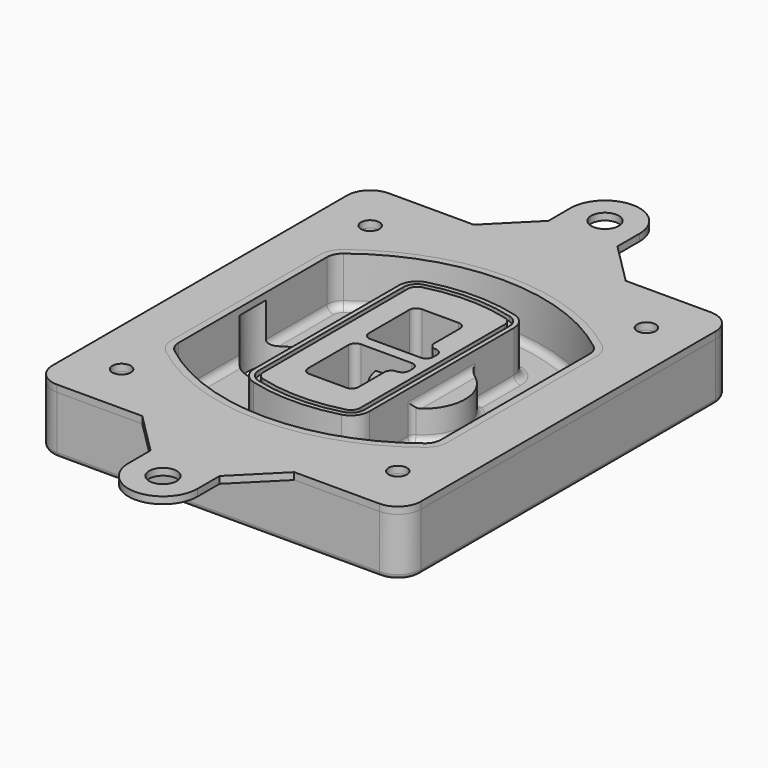
from build123d import *

# Parameters (mm, degrees)
F0_R      = 4
F1_DEPTH  = 25
F2_DEPTH  = 3
F3_DEPTH  = 18
F5_DEPTH  = 21
F6_DEPTH  = 2
F8_DEPTH  = 20
F9_DEPTH  = 16
F10_DEPTH = 25
F7_R      = 6
F7_R_2    = 4
F11_DEPTH = 6
F13_DEPTH = 9
F14_R     = 3
F15_R     = 2
F16_R     = 4
F16_R_2   = 6
F17_DEPTH = 3


with BuildPart() as f1:
    # F0 (on Top) → F1 (new body)
    with BuildSketch(Plane.XY):
        with BuildLine():
            ThreePointArc((-80, -80), (-77.0710678119, -87.0710678119), (-70, -90))
            Line((-70, -90), (70, -90))
            ThreePointArc((70, -90), (77.0710678119, -87.0710678119), (80, -80))
            Line((80, -80), (80, 80))
            ThreePointArc((80, 80), (77.0710678119, 87.0710678119), (70, 90))
            Line((70, 90), (-70, 90))
            ThreePointArc((-70, 90), (-77.0710678119, 87.0710678119), (-80, 80))
            Line((-80, 80), (-80, -80))
        make_face()
        with Locations((-60, -67.5)):
            Circle(F0_R, mode=Mode.SUBTRACT)
        with Locations((-60, 67.5)):
            Circle(F0_R, mode=Mode.SUBTRACT)
        with Locations((60, -67.5)):
            Circle(F0_R, mode=Mode.SUBTRACT)
        with BuildLine():
            ThreePointArc((-64, 40.2934422872), (-62.5820384798, 46.4328484224), (-58.6153846154, 51.3286200352))
            ThreePointArc((-58.6153846154, 51.3286200352), (0, 71.5), (58.6153846154, 51.3286200352))
            ThreePointArc((58.6153846154, 51.3286200352), (62.5820384798, 46.4328484224), (64, 40.2934422872))
            Line((64, 40.2934422872), (64, -40.2934422872))
            ThreePointArc((64, -40.2934422872), (62.5820384798, -46.4328484224), (58.6153846154, -51.3286200352))
            ThreePointArc((58.6153846154, -51.3286200352), (0, -71.5), (-58.6153846154, -51.3286200352))
            ThreePointArc((-58.6153846154, -51.3286200352), (-62.5820384798, -46.4328484224), (-64, -40.2934422872))
            Line((-64, -40.2934422872), (-64, 40.2934422872))
        make_face(mode=Mode.SUBTRACT)
        with Locations((60, 67.5)):
            Circle(F0_R, mode=Mode.SUBTRACT)
        with BuildLine():
            ThreePointArc((58.6153846154, 51.3286200352), (0, 71.5), (-58.6153846154, 51.3286200352))
            ThreePointArc((-58.6153846154, 51.3286200352), (-62.5820384798, 46.4328484224), (-64, 40.2934422872))
            Line((-64, 40.2934422872), (-64, -40.2934422872))
            ThreePointArc((-64, -40.2934422872), (-62.5820384798, -46.4328484224), (-58.6153846154, -51.3286200352))
            ThreePointArc((-58.6153846154, -51.3286200352), (0, -71.5), (58.6153846154, -51.3286200352))
            ThreePointArc((58.6153846154, -51.3286200352), (62.5820384798, -46.4328484224), (64, -40.2934422872))
            Line((64, -40.2934422872), (64, 40.2934422872))
            ThreePointArc((64, 40.2934422872), (62.5820384798, 46.4328484224), (58.6153846154, 51.3286200352))
        make_face()
        with BuildLine():
            Line((-60, -40.2934422872), (-60, 40.2934422872))
            ThreePointArc((-60, 40.2934422872), (-58.9871703427, 44.6787323838), (-56.1538461538, 48.1757121072))
            ThreePointArc((-56.1538461538, 48.1757121072), (0, 67.5), (56.1538461538, 48.1757121072))
            ThreePointArc((56.1538461538, 48.1757121072), (58.9871703427, 44.6787323838), (60, 40.2934422872))
            Line((60, 40.2934422872), (60, -40.2934422872))
            ThreePointArc((60, -40.2934422872), (58.9871703427, -44.6787323838), (56.1538461538, -48.1757121072))
            ThreePointArc((56.1538461538, -48.1757121072), (0, -67.5), (-56.1538461538, -48.1757121072))
            ThreePointArc((-56.1538461538, -48.1757121072), (-58.9871703427, -44.6787323838), (-60, -40.2934422872))
        make_face(mode=Mode.SUBTRACT)
        with BuildLine():
            ThreePointArc((-56.1538461538, 48.1757121072), (-58.9871703427, 44.6787323838), (-60, 40.2934422872))
            Line((-60, 40.2934422872), (-60, -40.2934422872))
            ThreePointArc((-60, -40.2934422872), (-58.9871703427, -44.6787323838), (-56.1538461538, -48.1757121072))
            ThreePointArc((-56.1538461538, -48.1757121072), (0, -67.5), (56.1538461538, -48.1757121072))
            ThreePointArc((56.1538461538, -48.1757121072), (58.9871703427, -44.6787323838), (60, -40.2934422872))
            Line((60, -40.2934422872), (60, 40.2934422872))
            ThreePointArc((60, 40.2934422872), (58.9871703427, 44.6787323838), (56.1538461538, 48.1757121072))
            ThreePointArc((56.1538461538, 48.1757121072), (0, 67.5), (-56.1538461538, 48.1757121072))
        make_face()
        with BuildLine():
            ThreePointArc((54.3076923077, 45.8110311612), (56.2910192399, 43.3631453548), (57, 40.2934422872))
            Line((57, 40.2934422872), (57, -40.2934422872))
            ThreePointArc((57, -40.2934422872), (56.2910192399, -43.3631453548), (54.3076923077, -45.8110311612))
            ThreePointArc((54.3076923077, -45.8110311612), (0, -64.5), (-54.3076923077, -45.8110311612))
            ThreePointArc((-54.3076923077, -45.8110311612), (-56.2910192399, -43.3631453548), (-57, -40.2934422872))
            Line((-57, -40.2934422872), (-57, 40.2934422872))
            ThreePointArc((-57, 40.2934422872), (-56.2910192399, 43.3631453548), (-54.3076923077, 45.8110311612))
            ThreePointArc((-54.3076923077, 45.8110311612), (0, 64.5), (54.3076923077, 45.8110311612))
        make_face(mode=Mode.SUBTRACT)
        with BuildLine():
            Line((57, -40.2934422872), (57, 40.2934422872))
            ThreePointArc((57, 40.2934422872), (56.2910192399, 43.3631453548), (54.3076923077, 45.8110311612))
            ThreePointArc((54.3076923077, 45.8110311612), (0, 64.5), (-54.3076923077, 45.8110311612))
            ThreePointArc((-54.3076923077, 45.8110311612), (-56.2910192399, 43.3631453548), (-57, 40.2934422872))
            Line((-57, 40.2934422872), (-57, -40.2934422872))
            ThreePointArc((-57, -40.2934422872), (-56.2910192399, -43.3631453548), (-54.3076923077, -45.8110311612))
            ThreePointArc((-54.3076923077, -45.8110311612), (0, -64.5), (54.3076923077, -45.8110311612))
            ThreePointArc((54.3076923077, -45.8110311612), (56.2910192399, -43.3631453548), (57, -40.2934422872))
        make_face()
    extrude(amount=-F1_DEPTH)

    # F0 (on Top) → F2 (join)
    with BuildSketch(Plane.XY):
        with BuildLine():
            ThreePointArc((-56.1538461538, 48.1757121072), (-58.9871703427, 44.6787323838), (-60, 40.2934422872))
            Line((-60, 40.2934422872), (-60, -40.2934422872))
            ThreePointArc((-60, -40.2934422872), (-58.9871703427, -44.6787323838), (-56.1538461538, -48.1757121072))
            ThreePointArc((-56.1538461538, -48.1757121072), (0, -67.5), (56.1538461538, -48.1757121072))
            ThreePointArc((56.1538461538, -48.1757121072), (58.9871703427, -44.6787323838), (60, -40.2934422872))
            Line((60, -40.2934422872), (60, 40.2934422872))
            ThreePointArc((60, 40.2934422872), (58.9871703427, 44.6787323838), (56.1538461538, 48.1757121072))
            ThreePointArc((56.1538461538, 48.1757121072), (0, 67.5), (-56.1538461538, 48.1757121072))
        make_face()
        with BuildLine():
            ThreePointArc((54.3076923077, 45.8110311612), (56.2910192399, 43.3631453548), (57, 40.2934422872))
            Line((57, 40.2934422872), (57, -40.2934422872))
            ThreePointArc((57, -40.2934422872), (56.2910192399, -43.3631453548), (54.3076923077, -45.8110311612))
            ThreePointArc((54.3076923077, -45.8110311612), (0, -64.5), (-54.3076923077, -45.8110311612))
            ThreePointArc((-54.3076923077, -45.8110311612), (-56.2910192399, -43.3631453548), (-57, -40.2934422872))
            Line((-57, -40.2934422872), (-57, 40.2934422872))
            ThreePointArc((-57, 40.2934422872), (-56.2910192399, 43.3631453548), (-54.3076923077, 45.8110311612))
            ThreePointArc((-54.3076923077, 45.8110311612), (0, 64.5), (54.3076923077, 45.8110311612))
        make_face(mode=Mode.SUBTRACT)
    extrude(amount=F2_DEPTH)

    # F0 (on Top) → F3 (cut)
    with BuildSketch(Plane.XY):
        with BuildLine():
            Line((57, -40.2934422872), (57, 40.2934422872))
            ThreePointArc((57, 40.2934422872), (56.2910192399, 43.3631453548), (54.3076923077, 45.8110311612))
            ThreePointArc((54.3076923077, 45.8110311612), (0, 64.5), (-54.3076923077, 45.8110311612))
            ThreePointArc((-54.3076923077, 45.8110311612), (-56.2910192399, 43.3631453548), (-57, 40.2934422872))
            Line((-57, 40.2934422872), (-57, -40.2934422872))
            ThreePointArc((-57, -40.2934422872), (-56.2910192399, -43.3631453548), (-54.3076923077, -45.8110311612))
            ThreePointArc((-54.3076923077, -45.8110311612), (0, -64.5), (54.3076923077, -45.8110311612))
            ThreePointArc((54.3076923077, -45.8110311612), (56.2910192399, -43.3631453548), (57, -40.2934422872))
        make_face()
    extrude(amount=-F3_DEPTH, mode=Mode.SUBTRACT)

    # F4 (on face) → F5 (join, through all)
    with BuildSketch(Plane.XY.offset(3)):
        with BuildLine():
            ThreePointArc((-25, -39.2465276821), (-23.3511545998, -44.1109737193), (-19.0842911877, -46.9702398883))
            ThreePointArc((-19.0842911877, -46.9702398883), (0, -49.5), (19.0842911877, -46.9702398883))
            ThreePointArc((19.0842911877, -46.9702398883), (23.3511545998, -44.1109737193), (25, -39.2465276821))
            Line((25, -39.2465276821), (25, 39.2465276821))
            ThreePointArc((25, 39.2465276821), (23.3511545998, 44.1109737193), (19.0842911877, 46.9702398883))
            ThreePointArc((19.0842911877, 46.9702398883), (0, 49.5), (-19.0842911877, 46.9702398883))
            ThreePointArc((-19.0842911877, 46.9702398883), (-23.3511545998, 44.1109737193), (-25, 39.2465276821))
            Line((-25, 39.2465276821), (-25, -39.2465276821))
        make_face()
        with BuildLine():
            ThreePointArc((18.5632183908, 45.0393118368), (21.7633659499, 42.89486221), (23, 39.2465276821))
            Line((23, 39.2465276821), (23, -39.2465276821))
            ThreePointArc((23, -39.2465276821), (21.7633659499, -42.89486221), (18.5632183908, -45.0393118368))
            ThreePointArc((18.5632183908, -45.0393118368), (0, -47.5), (-18.5632183908, -45.0393118368))
            ThreePointArc((-18.5632183908, -45.0393118368), (-21.7633659499, -42.89486221), (-23, -39.2465276821))
            Line((-23, -39.2465276821), (-23, 39.2465276821))
            ThreePointArc((-23, 39.2465276821), (-21.7633659499, 42.89486221), (-18.5632183908, 45.0393118368))
            ThreePointArc((-18.5632183908, 45.0393118368), (0, 47.5), (18.5632183908, 45.0393118368))
        make_face(mode=Mode.SUBTRACT)
        with BuildLine():
            Line((23, -39.2465276821), (23, 39.2465276821))
            ThreePointArc((23, 39.2465276821), (21.7633659499, 42.89486221), (18.5632183908, 45.0393118368))
            ThreePointArc((18.5632183908, 45.0393118368), (0, 47.5), (-18.5632183908, 45.0393118368))
            ThreePointArc((-18.5632183908, 45.0393118368), (-21.7633659499, 42.89486221), (-23, 39.2465276821))
            Line((-23, 39.2465276821), (-23, -39.2465276821))
            ThreePointArc((-23, -39.2465276821), (-21.7633659499, -42.89486221), (-18.5632183908, -45.0393118368))
            ThreePointArc((-18.5632183908, -45.0393118368), (0, -47.5), (18.5632183908, -45.0393118368))
            ThreePointArc((18.5632183908, -45.0393118368), (21.7633659499, -42.89486221), (23, -39.2465276821))
        make_face()
        with BuildLine():
            ThreePointArc((18.0421455939, 43.1083837852), (20.1755772999, 41.6787507007), (21, 39.2465276821))
            Line((21, 39.2465276821), (21, -39.2465276821))
            ThreePointArc((21, -39.2465276821), (20.1755772999, -41.6787507007), (18.0421455939, -43.1083837852))
            ThreePointArc((18.0421455939, -43.1083837852), (0, -45.5), (-18.0421455939, -43.1083837852))
            ThreePointArc((-18.0421455939, -43.1083837852), (-20.1755772999, -41.6787507007), (-21, -39.2465276821))
            Line((-21, -39.2465276821), (-21, 39.2465276821))
            ThreePointArc((-21, 39.2465276821), (-20.1755772999, 41.6787507007), (-18.0421455939, 43.1083837852))
            ThreePointArc((-18.0421455939, 43.1083837852), (0, 45.5), (18.0421455939, 43.1083837852))
        make_face(mode=Mode.SUBTRACT)
        with BuildLine():
            Line((21, -39.2465276821), (21, 39.2465276821))
            ThreePointArc((21, 39.2465276821), (20.1755772999, 41.6787507007), (18.0421455939, 43.1083837852))
            ThreePointArc((18.0421455939, 43.1083837852), (0, 45.5), (-18.0421455939, 43.1083837852))
            ThreePointArc((-18.0421455939, 43.1083837852), (-20.1755772999, 41.6787507007), (-21, 39.2465276821))
            Line((-21, 39.2465276821), (-21, -39.2465276821))
            ThreePointArc((-21, -39.2465276821), (-20.1755772999, -41.6787507007), (-18.0421455939, -43.1083837852))
            ThreePointArc((-18.0421455939, -43.1083837852), (0, -45.5), (18.0421455939, -43.1083837852))
            ThreePointArc((18.0421455939, -43.1083837852), (20.1755772999, -41.6787507007), (21, -39.2465276821))
        make_face()
        with BuildLine():
            Line((-8, -2.5), (14, -2.5))
            ThreePointArc((14, -2.5), (16.1213203436, -3.3786796564), (17, -5.5))
            Line((17, -5.5), (17, -7.5))
            ThreePointArc((17, -7.5), (16.1213203436, -9.6213203436), (14, -10.5))
            ThreePointArc((14, -10.5), (11.8786796564, -11.3786796564), (11, -13.5))
            Line((11, -13.5), (11, -27.5))
            ThreePointArc((11, -27.5), (10.1213203436, -29.6213203436), (8, -30.5))
            Line((8, -30.5), (-8, -30.5))
            ThreePointArc((-8, -30.5), (-10.1213203436, -29.6213203436), (-11, -27.5))
            Line((-11, -27.5), (-11, -5.5))
            ThreePointArc((-11, -5.5), (-10.1213203436, -3.3786796564), (-8, -2.5))
        make_face(mode=Mode.SUBTRACT)
        with BuildLine():
            ThreePointArc((-8, 2.5), (-10.1213203436, 3.3786796564), (-11, 5.5))
            Line((-11, 5.5), (-11, 27.5))
            ThreePointArc((-11, 27.5), (-10.1213203436, 29.6213203436), (-8, 30.5))
            Line((-8, 30.5), (8, 30.5))
            ThreePointArc((8, 30.5), (10.1213203436, 29.6213203436), (11, 27.5))
            Line((11, 27.5), (11, 13.5))
            ThreePointArc((11, 13.5), (11.8786796564, 11.3786796564), (14, 10.5))
            ThreePointArc((14, 10.5), (16.1213203436, 9.6213203436), (17, 7.5))
            Line((17, 7.5), (17, 5.5))
            ThreePointArc((17, 5.5), (16.1213203436, 3.3786796564), (14, 2.5))
            Line((14, 2.5), (-8, 2.5))
        make_face(mode=Mode.SUBTRACT)
    extrude(amount=-F5_DEPTH)

    # F4 (on face) → F6 (cut)
    with BuildSketch(Plane.XY.offset(3)):
        with BuildLine():
            Line((23, -39.2465276821), (23, 39.2465276821))
            ThreePointArc((23, 39.2465276821), (21.7633659499, 42.89486221), (18.5632183908, 45.0393118368))
            ThreePointArc((18.5632183908, 45.0393118368), (0, 47.5), (-18.5632183908, 45.0393118368))
            ThreePointArc((-18.5632183908, 45.0393118368), (-21.7633659499, 42.89486221), (-23, 39.2465276821))
            Line((-23, 39.2465276821), (-23, -39.2465276821))
            ThreePointArc((-23, -39.2465276821), (-21.7633659499, -42.89486221), (-18.5632183908, -45.0393118368))
            ThreePointArc((-18.5632183908, -45.0393118368), (0, -47.5), (18.5632183908, -45.0393118368))
            ThreePointArc((18.5632183908, -45.0393118368), (21.7633659499, -42.89486221), (23, -39.2465276821))
        make_face()
        with BuildLine():
            ThreePointArc((18.0421455939, 43.1083837852), (20.1755772999, 41.6787507007), (21, 39.2465276821))
            Line((21, 39.2465276821), (21, -39.2465276821))
            ThreePointArc((21, -39.2465276821), (20.1755772999, -41.6787507007), (18.0421455939, -43.1083837852))
            ThreePointArc((18.0421455939, -43.1083837852), (0, -45.5), (-18.0421455939, -43.1083837852))
            ThreePointArc((-18.0421455939, -43.1083837852), (-20.1755772999, -41.6787507007), (-21, -39.2465276821))
            Line((-21, -39.2465276821), (-21, 39.2465276821))
            ThreePointArc((-21, 39.2465276821), (-20.1755772999, 41.6787507007), (-18.0421455939, 43.1083837852))
            ThreePointArc((-18.0421455939, 43.1083837852), (0, 45.5), (18.0421455939, 43.1083837852))
        make_face(mode=Mode.SUBTRACT)
    extrude(amount=-F6_DEPTH, mode=Mode.SUBTRACT)

    # F7 (on face) → F8 (join)
    with BuildSketch(Plane(origin=(0, 0, -25), x_dir=(1, 0, 0), z_dir=(0, 0, -1))):
        with BuildLine():
            ThreePointArc((3.28842436, 0), (16.7567035675, 13.4682792075), (30.224982775, 0))
            Line((30.224982775, 0), (35.224982775, 0))
            ThreePointArc((35.224982775, 0), (16.7567035675, 18.4682792075), (-1.71157564, 0))
            Line((-1.71157564, 0), (3.28842436, 0))
        make_face()
        with BuildLine():
            Line((3.28842436, 0), (30.224982775, 0))
            ThreePointArc((30.224982775, 0), (16.7567035675, 13.4682792075), (3.28842436, 0))
        make_face()
        with BuildLine():
            ThreePointArc((3.28842436, 0), (16.7567035675, -13.4682792075), (30.224982775, 0))
            Line((30.224982775, 0), (3.28842436, 0))
        make_face()
        with BuildLine():
            Line((35.224982775, 0), (30.224982775, 0))
            ThreePointArc((30.224982775, 0), (16.7567035675, -13.4682792075), (3.28842436, 0))
            Line((3.28842436, 0), (-1.71157564, 0))
            ThreePointArc((-1.71157564, 0), (16.7567035675, -18.4682792075), (35.224982775, 0))
        make_face()
    extrude(amount=-F8_DEPTH)

    # F7 (on face) → F9 (cut)
    with BuildSketch(Plane(origin=(0, 0, -25), x_dir=(1, 0, 0), z_dir=(0, 0, -1))):
        with BuildLine():
            Line((3.28842436, 0), (30.224982775, 0))
            ThreePointArc((30.224982775, 0), (16.7567035675, 13.4682792075), (3.28842436, 0))
        make_face()
        with BuildLine():
            ThreePointArc((3.28842436, 0), (16.7567035675, -13.4682792075), (30.224982775, 0))
            Line((30.224982775, 0), (3.28842436, 0))
        make_face()
    extrude(amount=-F9_DEPTH, mode=Mode.SUBTRACT)

    # F7 (on face) → F10 (cut)
    with BuildSketch(Plane(origin=(0, 0, -25), x_dir=(1, 0, 0), z_dir=(0, 0, -1))):
        with BuildLine():
            Line((-59.0318229325, 0), (-32.0952645175, 0))
            ThreePointArc((-32.0952645175, 0), (-45.563543725, 13.4682792075), (-59.0318229325, 0))
        make_face()
        with BuildLine():
            ThreePointArc((-59.0318229325, 0), (-45.563543725, -13.4682792075), (-32.0952645175, 0))
            Line((-32.0952645175, 0), (-59.0318229325, 0))
        make_face()
    extrude(amount=-F10_DEPTH, mode=Mode.SUBTRACT)

    # F7 (on face) → F11 (cut)
    with BuildSketch(Plane(origin=(0, 0, -25), x_dir=(1, 0, 0), z_dir=(0, 0, -1))):
        with Locations((60, -67.5)):
            Circle(F7_R)
        with Locations((60, -67.5)):
            Circle(F7_R_2, mode=Mode.SUBTRACT)
        with Locations((-60, -67.5)):
            Circle(F7_R)
        with Locations((-60, -67.5)):
            Circle(F7_R_2, mode=Mode.SUBTRACT)
        with Locations((-60, 67.5)):
            Circle(F7_R)
        with Locations((-60, 67.5)):
            Circle(F7_R_2, mode=Mode.SUBTRACT)
        with Locations((60, 67.5)):
            Circle(F7_R)
        with Locations((60, 67.5)):
            Circle(F7_R_2, mode=Mode.SUBTRACT)
    extrude(amount=-F11_DEPTH, mode=Mode.SUBTRACT)

    # F12 (on face) → F13 (cut, through all)
    with BuildSketch(Plane(origin=(0, 0, -9), x_dir=(1, 0, 0), z_dir=(0, 0, -1))):
        with BuildLine():
            Line((11, 13.5), (11, 17.5481537753))
            ThreePointArc((11, 17.5481537753), (2.5696536419, 11.8239143813), (-1.5415842455, 2.5))
            Line((-1.5415842455, 2.5), (3.5224848595, 2.5))
            ThreePointArc((3.5224848595, 2.5), (6.1857188154, 8.3455872281), (11.2536447004, 12.2927168648))
            ThreePointArc((11.2536447004, 12.2927168648), (11.0640958889, 12.8831798879), (11, 13.5))
        make_face()
        with BuildLine():
            ThreePointArc((11.2536447004, -12.2927168648), (6.1857188154, -8.3455872281), (3.5224848595, -2.5))
            Line((3.5224848595, -2.5), (-1.5415842455, -2.5))
            ThreePointArc((-1.5415842455, -2.5), (2.5696536419, -11.8239143813), (11, -17.5481537753))
            Line((11, -17.5481537753), (11, -13.5))
            ThreePointArc((11, -13.5), (11.0640958889, -12.8831798879), (11.2536447004, -12.2927168648))
        make_face()
        with BuildLine():
            ThreePointArc((11.2536447004, 12.2927168648), (6.1857188154, 8.3455872281), (3.5224848595, 2.5))
            Line((3.5224848595, 2.5), (14, 2.5))
            ThreePointArc((14, 2.5), (16.1213203436, 3.3786796564), (17, 5.5))
            Line((17, 5.5), (17, 7.5))
            ThreePointArc((17, 7.5), (16.1213203436, 9.6213203436), (14, 10.5))
            ThreePointArc((14, 10.5), (12.3601599782, 10.9878446101), (11.2536447004, 12.2927168648))
        make_face()
        with BuildLine():
            Line((14, -2.5), (3.5224848595, -2.5))
            ThreePointArc((3.5224848595, -2.5), (6.1857188154, -8.3455872281), (11.2536447004, -12.2927168648))
            ThreePointArc((11.2536447004, -12.2927168648), (12.3601599782, -10.9878446101), (14, -10.5))
            ThreePointArc((14, -10.5), (16.1213203436, -9.6213203436), (17, -7.5))
            Line((17, -7.5), (17, -5.5))
            ThreePointArc((17, -5.5), (16.1213203436, -3.3786796564), (14, -2.5))
        make_face()
    extrude(amount=F13_DEPTH, mode=Mode.SUBTRACT)

    # F14
    f14_edges = [f1.edges().sort_by_distance(p)[0] for p in [
        (-57, -23.703476, -18),
        (-57, 23.703476, -18),
        (25, 0, -5),
        (25, 16.526506, -11.5),
        (25, -16.526506, -11.5),
        (25, -27.886517, -18),
        (35.224983, 0, -18),
    ]]
    fillet(f14_edges, radius=F14_R)

    # F15
    f15_edges = [f1.edges().sort_by_distance(p)[0] for p in [
        (0, -90, -25),
    ]]
    fillet(f15_edges, radius=F15_R)


with BuildPart() as f17:
    # F16 (on Top) → F17 (new body, through all)
    with BuildSketch(Plane.XY):
        with BuildLine():
            Line((-33, 90), (-70, 90))
            ThreePointArc((-70, 90), (-77.0710678119, 87.0710678119), (-80, 80))
            Line((-80, 80), (-80, -80))
            ThreePointArc((-80, -80), (-77.0710678119, -87.0710678119), (-70, -90))
            Line((-70, -90), (-33, -90))
            Line((-33, -90), (33, -90))
            Line((33, -90), (70, -90))
            ThreePointArc((70, -90), (77.0710678119, -87.0710678119), (80, -80))
            Line((80, -80), (80, 80))
            ThreePointArc((80, 80), (77.0710678119, 87.0710678119), (70, 90))
            Line((70, 90), (33, 90))
            Line((33, 90), (-33, 90))
        make_face()
        with Locations((-60, -67.5)):
            Circle(F16_R, mode=Mode.SUBTRACT)
        with Locations((60, -67.5)):
            Circle(F16_R, mode=Mode.SUBTRACT)
        with Locations((-60, 67.5)):
            Circle(F16_R, mode=Mode.SUBTRACT)
        with BuildLine():
            Line((-60, -40.2934422872), (-60, 40.2934422872))
            ThreePointArc((-60, 40.2934422872), (-58.9871703427, 44.6787323838), (-56.1538461538, 48.1757121072))
            ThreePointArc((-56.1538461538, 48.1757121072), (0, 67.5), (56.1538461538, 48.1757121072))
            ThreePointArc((56.1538461538, 48.1757121072), (58.9871703427, 44.6787323838), (60, 40.2934422872))
            Line((60, 40.2934422872), (60, -40.2934422872))
            ThreePointArc((60, -40.2934422872), (58.9871703427, -44.6787323838), (56.1538461538, -48.1757121072))
            ThreePointArc((56.1538461538, -48.1757121072), (0, -67.5), (-56.1538461538, -48.1757121072))
            ThreePointArc((-56.1538461538, -48.1757121072), (-58.9871703427, -44.6787323838), (-60, -40.2934422872))
        make_face(mode=Mode.SUBTRACT)
        with Locations((60, 67.5)):
            Circle(F16_R, mode=Mode.SUBTRACT)
        with BuildLine():
            Line((-15, 108), (-33, 90))
            Line((-33, 90), (33, 90))
            Line((33, 90), (15, 108))
            Line((15, 108), (15, 120))
            ThreePointArc((15, 120), (0, 135), (-15, 120))
            Line((-15, 120), (-15, 108))
        make_face()
        with Locations((0, 120)):
            Circle(F16_R_2, mode=Mode.SUBTRACT)
        with BuildLine():
            Line((33, -90), (-33, -90))
            Line((-33, -90), (-15, -108))
            Line((-15, -108), (-15, -120))
            ThreePointArc((-15, -120), (0, -135), (15, -120))
            Line((15, -120), (15, -108))
            Line((15, -108), (33, -90))
        make_face()
        with Locations((0, -120)):
            Circle(F16_R_2, mode=Mode.SUBTRACT)
    extrude(amount=F17_DEPTH)


solid = Compound([f1.part, f17.part])
